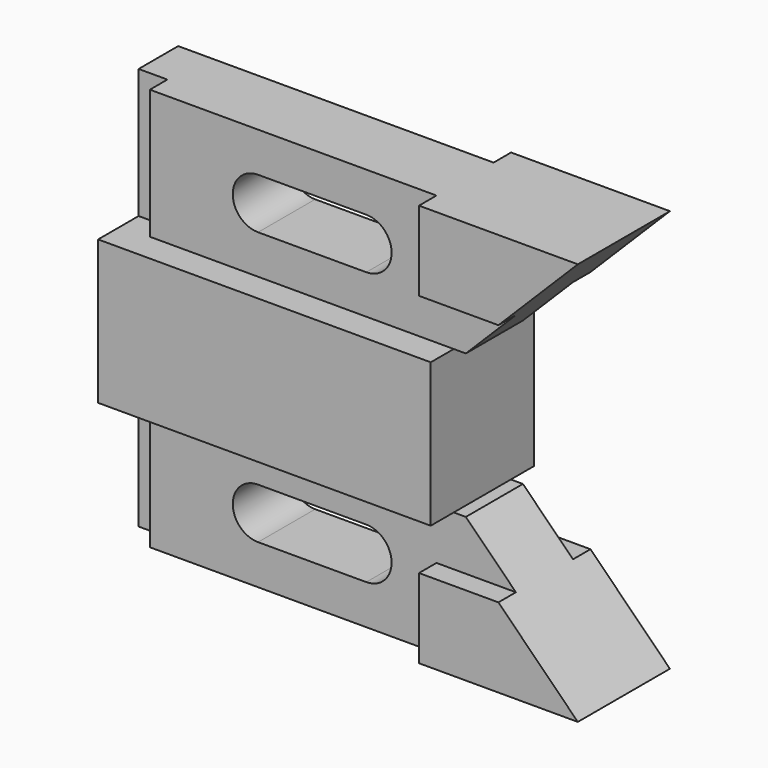
from build123d import *

# Parameters (mm, degrees)
F1_DEPTH = 104.648
F3_DEPTH = 28.449
F5_W     = 69.596
F5_H     = 4.826
F6_DEPTH = 28.575
F8_DEPTH = 22.099


# Not quite as in the source:
# - a pattern or mirror of a feature is missing from the dataset's text; its kind, count and spacing are read off the source's solid


with BuildPart() as f1:
    # F0 (on Right) → F1 (new body)
    with BuildSketch(Plane.YZ):
        Polygon((12.7, 44.45), (0, 44.45), (-12.7, 44.45), (-12.7, 26.924), (-7.874, 26.924), (-7.874, 15.875), (-14.224, 15.875), (-14.224, 0), (-14.224, -15.875), (-7.874, -15.875), (-7.874, -26.924), (-12.7, -26.924), (-12.7, -44.45), (0, -44.45), (12.7, -44.45), (12.7, -26.924), (7.874, -26.924), (7.874, -15.875), (14.224, -15.875), (14.224, 0), (14.224, 15.875), (7.874, 15.875), (7.874, 26.924), (12.7, 26.924), align=None)
    extrude(amount=F1_DEPTH)

    # F2 (on face) → F3 (cut, through all)
    with BuildSketch(Plane.XZ.offset(14.224)):
        Polygon((73.406, 15.875), (73.406, 0), (73.406, -15.875), (76.073, -15.875), (104.648, -44.45), (104.648, -15.875), (104.648, 0), (104.648, 15.875), (104.648, 44.45), (76.073, 15.875), align=None)
    extrude(amount=-F3_DEPTH, mode=Mode.SUBTRACT)

    # F5 (on face) → F6 (cut)
    with BuildSketch(Plane.XY.offset(44.45)):
        with Locations((34.798, 10.287)):
            Rectangle(F5_W, F5_H)
        Polygon((0, -3.048), (0, -12.7), (69.596, -12.7), (69.596, -7.874), (6.35, -7.874), (6.35, -3.048), align=None)
    f6 = extrude(amount=-F6_DEPTH, mode=Mode.SUBTRACT)

    # F6_copies: F6 across plane
    add(f6.mirror(Plane(origin=(0, 0, 0), x_dir=(-1, 0, 0), z_dir=(0, 0, -1))), mode=Mode.SUBTRACT)

    # F7 (on face) → F8 (cut, through all)
    with BuildSketch(Plane.XZ.offset(7.874)):
        with BuildLine():
            Line((42.164, 35.687), (30.226, 35.687))
            ThreePointArc((30.226, 35.687), (24.638, 30.099), (30.226, 24.511))
            Line((30.226, 24.511), (42.164, 24.511))
            Line((42.164, 24.511), (54.102, 24.511))
            ThreePointArc((54.102, 24.511), (59.69, 30.099), (54.102, 35.687))
            Line((54.102, 35.687), (42.164, 35.687))
        make_face()
    f8 = extrude(amount=-F8_DEPTH, mode=Mode.SUBTRACT)

    # F8_copies: F8 across plane
    add(f8.mirror(Plane(origin=(0, 0, 0), x_dir=(-1, 0, 0), z_dir=(0, 0, -1))), mode=Mode.SUBTRACT)


solid = f1.part
